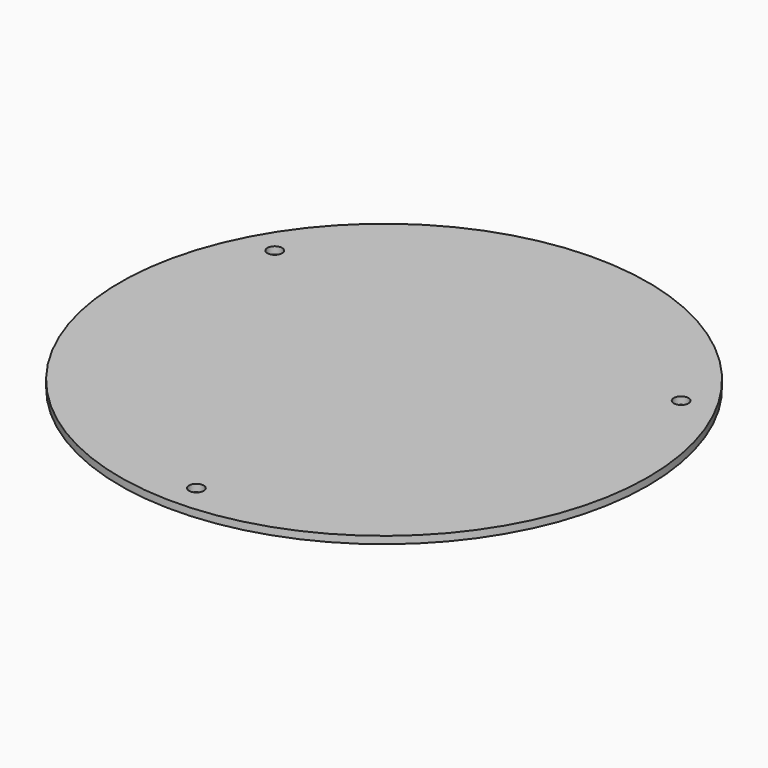
from build123d import *

# Parameters (mm, degrees)
F0_R     = 114.3
F0_R_2   = 3.175
F1_DEPTH = 3.175


# Not quite as in the source:
# - a feature names something its author has since deleted; it is built from what else it names


with BuildPart() as f1:
    # F0 (on Top) → F1 (new body)
    with BuildSketch(Plane.XY):
        Circle(F0_R)
        with Locations((0, -101.6)):
            Circle(F0_R_2, mode=Mode.SUBTRACT)
        with Locations((-87.9881810245, 50.8)):
            Circle(F0_R_2, mode=Mode.SUBTRACT)
        with Locations((87.9881810245, 50.8)):
            Circle(F0_R_2, mode=Mode.SUBTRACT)
    extrude(amount=F1_DEPTH)


solid = f1.part
